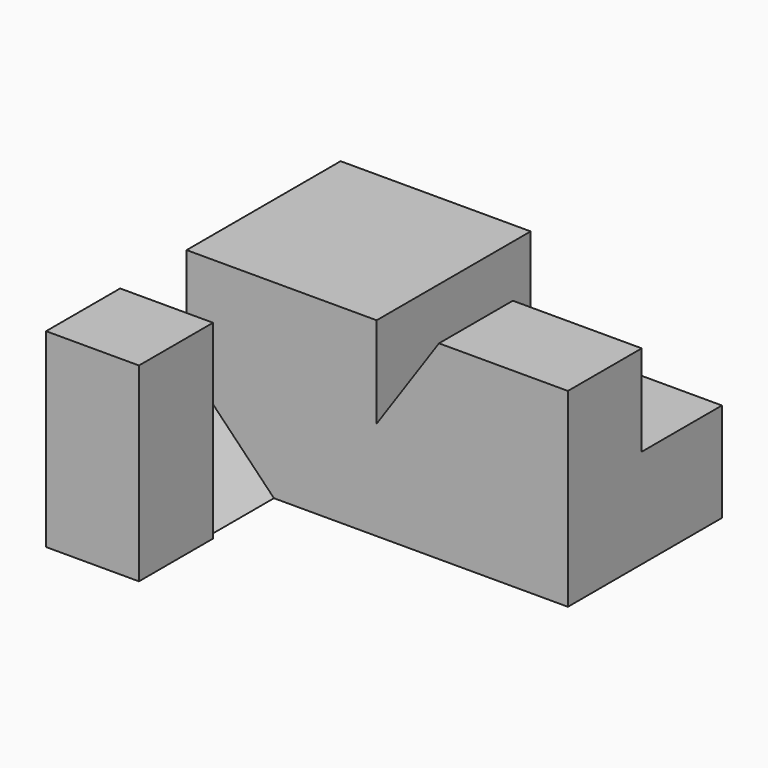
from build123d import *

# Parameters (mm, degrees)
F0_W     = 15.748
F0_H     = 15.748
F1_DEPTH = 15.9512
F3_DEPTH = 6.8834
F5_DEPTH = 7.6708
F6_W     = 15.9512
F6_H     = 8.2042
F7_DEPTH = 15.8496
F9_DEPTH = 7.6454


with BuildPart() as f1:
    # F0 (on Front) → F1 (new body)
    with BuildSketch(Plane.XZ):
        with Locations((7.874, 7.874)):
            Rectangle(F0_W, F0_H)
    extrude(amount=F1_DEPTH)

    # F2 (on face) → F3 (join)
    with BuildSketch(Plane.XZ.offset(15.9512)):
        Polygon((0, 7.4676), (0, 0), (7.239, 0), align=None)
    extrude(amount=F3_DEPTH)

    # F4 (on face) → F5 (join)
    with BuildSketch(Plane.XZ.offset(22.8346)):
        Polygon((0, 7.4676), (7.239, 0), (7.6962, 0), (7.6962, 15.748), (0, 15.748), align=None)
        Polygon((0, 7.4676), (0, 0), (7.239, 0), align=None)
    extrude(amount=F5_DEPTH)

    # F6 (on face) → F7 (join)
    with BuildSketch(Plane.YZ.offset(15.748)):
        with Locations((-7.9756, 4.1021)):
            Rectangle(F6_W, F6_H)
    extrude(amount=F7_DEPTH)

    # F8 (on face) → F9 (join)
    with BuildSketch(Plane.XZ.offset(15.9512)):
        Polygon((20.9155736628, 15.748), (15.748, 8.2042), (31.5976, 8.2042), (31.5976, 15.748), align=None)
    extrude(amount=-F9_DEPTH)


solid = f1.part
